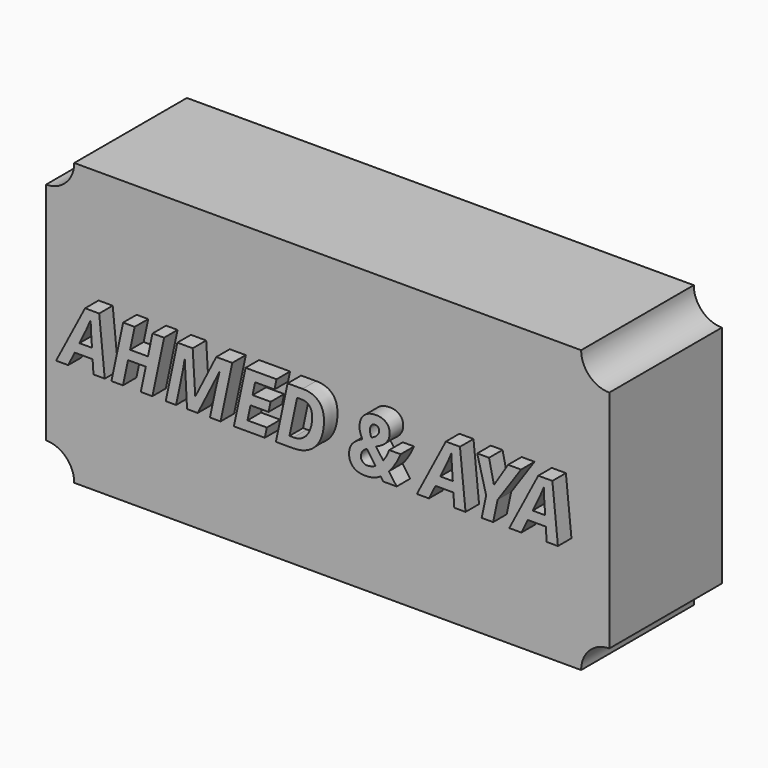
from build123d import *

# Parameters (mm, degrees)
F1_DEPTH     = 25
F2_TEXT_SIZE = 13.7637697436
F3_DEPTH     = 3


# Not quite as in the source:
# - Text() gives the source's letters only with a copy of the font that has no kerning and outlines rounded to 1/6400 em; it was checked with that copy


with BuildPart() as f1:
    # F0 (on Front) → F1 (new body)
    with BuildSketch(Plane.XZ):
        with BuildLine():
            ThreePointArc((50, 20), (46.4644660941, 21.4644660941), (45, 25))
            Line((45, 25), (-45, 25))
            ThreePointArc((-45, 25), (-46.4644660941, 21.4644660941), (-50, 20))
            Line((-50, 20), (-50, -20))
            ThreePointArc((-50, -20), (-46.4644660941, -21.4644660941), (-45, -25))
            Line((-45, -25), (45, -25))
            ThreePointArc((45, -25), (46.4644660941, -21.4644660941), (50, -20))
            Line((50, -20), (50, 20))
        make_face()
    extrude(amount=-F1_DEPTH)

    # F2 (on Front) → F3 (join)
    with BuildSketch(Plane.XZ):
        with Locations((-45, -4.955)):
            Text('AHMED & AYA', F2_TEXT_SIZE, font='Open Sans', font_style=FontStyle.BOLDITALIC, text_align=(TextAlign.LEFT, TextAlign.BOTTOM))
    extrude(amount=F3_DEPTH)


solid = f1.part
